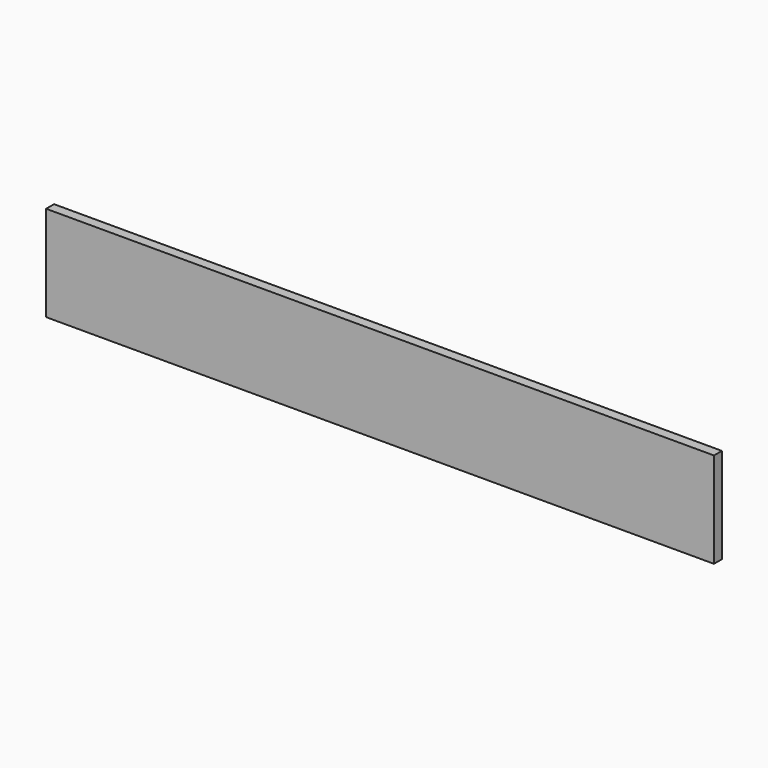
from build123d import *

# Parameters (mm, degrees)
F0_W     = 1066.8
F0_H     = 152.4
F1_DEPTH = 15.875


# Not quite as in the source:
# - a length typed as a fraction of an inch, garbled in the dataset ("3 / 203.2 mm" for 3/8 in), is restored


with BuildPart() as f1:
    # F0 (on Front) → F1 (new body)
    with BuildSketch(Plane.XZ):
        with Locations((533.4, 76.2)):
            Rectangle(F0_W, F0_H)
    extrude(amount=F1_DEPTH)


solid = f1.part
